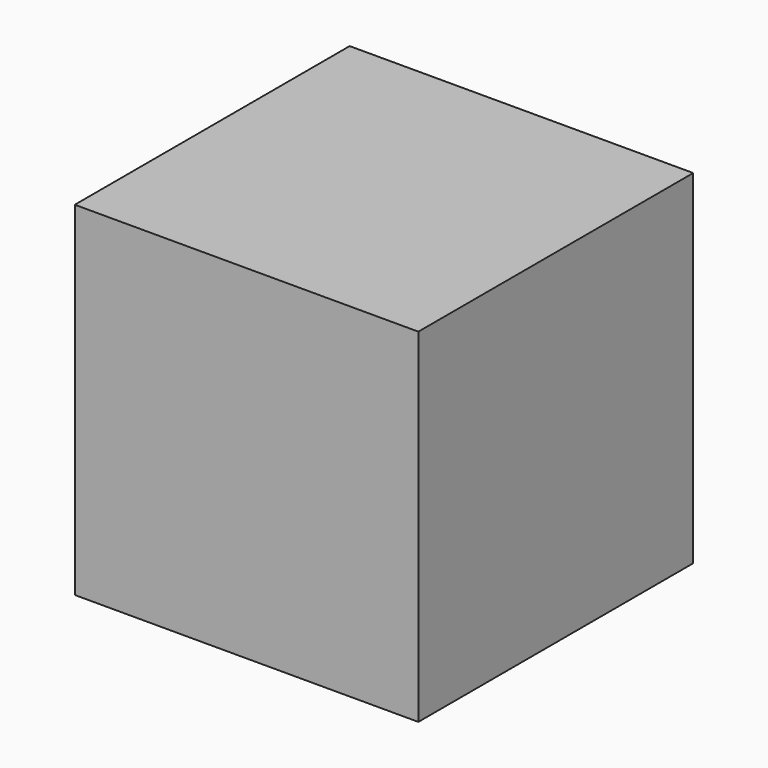
from build123d import *
from build123d import SkipClean  # not in build123d's __all__

# Parameters (mm, degrees)
F0_W     = 40
F0_H     = 40
F1_DEPTH = 40


with BuildPart() as f1:
    # F0 (on Front) → F1 (new body)
    with BuildSketch(Plane.XZ):
        with Locations((-20, 20)):
            Rectangle(F0_W, F0_H)
    extrude(amount=F1_DEPTH)

    # F2 (on face) → F3 (revolve)
    with BuildSketch(Plane(origin=(0, 0, 0), x_dir=(-1, 0, 0), z_dir=(0, 1, 0))):
        with BuildLine():
            ThreePointArc((12.5309191644, 0), (21.2226156145, -7.0983319264), (29.9143120646, 0))
            Line((29.9143120646, 0), (12.5309191644, 0))
        make_face()
    with SkipClean():  # cleaning this boolean's faces spoils the solid; the shape is the same uncleaned
        revolve(axis=Axis((-21.2226156145, 0, 0), (1, 0, 0)))


solid = f1.part
